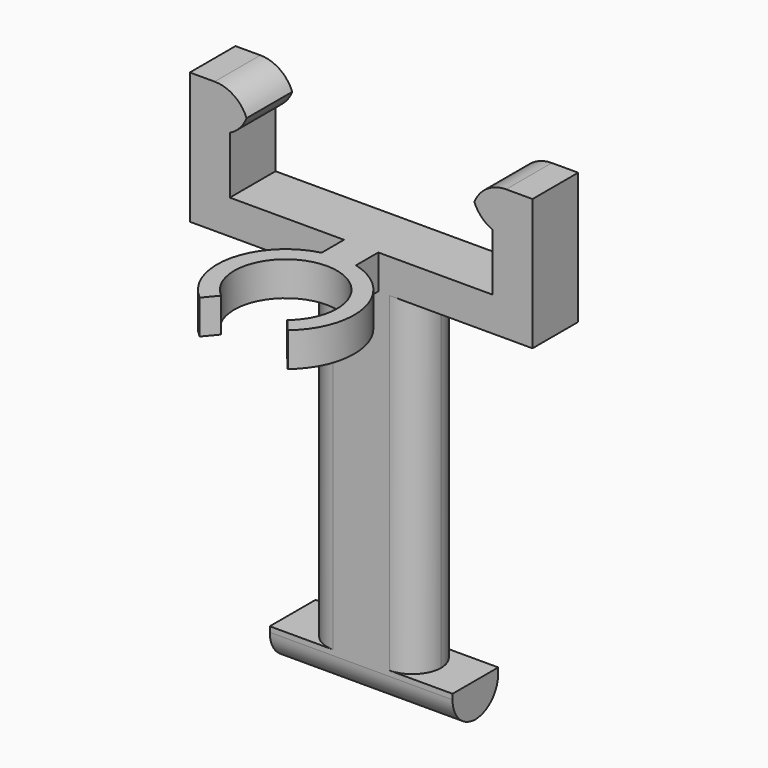
from build123d import *

# Parameters (mm, degrees)
F1_DEPTH    = 3
F3_DEPTH    = 5
F4_T1_DEPTH = 20
F4_T3_DEPTH = 18.7590602534
F4_T5_DEPTH = 18.4414894703
F5_T1_DEPTH = 28.8976125792
F5_T3_DEPTH = 28.7


# Not quite as in the source:
# - a fillet or chamfer that OpenCascade refuses, or shapes differently, is made with other operations: its cross-section is extruded or revolved along the edge and cut away or added


with BuildPart() as f1:
    # F0 (on Top) → F1 (new body)
    with BuildSketch(Plane.XY):
        with BuildLine():
            ThreePointArc((-2.8925442436, -3.447199994), (0, 4.5), (2.8925442436, -3.447199994))
            Line((2.8925442436, -3.447199994), (3.8567256581, -4.5962666587))
            ThreePointArc((3.8567256581, -4.5962666587), (5.9714768944, 0.5843489538), (2.8925442436, 5.2567278605))
            ThreePointArc((2.8925442436, 5.2567278605), (2.2135929139, 5.5767379723), (1.5, 5.8094750193))
            Line((1.5, 5.8094750193), (1.5, 8.2567278605))
            Line((1.5, 8.2567278605), (-1.5, 8.2567278605))
            Line((-1.5, 8.2567278605), (-1.5, 5.8094750193))
            ThreePointArc((-1.5, 5.8094750193), (-5.8517939481, 1.3253330104), (-3.8567256581, -4.5962666587))
            Line((-3.8567256581, -4.5962666587), (-2.8925442436, -3.447199994))
        make_face()
    extrude(amount=F1_DEPTH)

    # F2 (on face) → F3 (join)
    with BuildSketch(Plane(origin=(0, 8.2567278605, 0), x_dir=(-1, 0, 0), z_dir=(0, 1, 0))):
        Polygon((-15, 0), (-5, 0), (-5, -28.8976125792), (-8, -28.8976125792), (-8, -31.8976125792), (8, -31.8976125792), (8, -28.8976125792), (5, -28.8976125792), (5, 0), (15, 0), (15, 3), (15, 8), (15, 11.5052), (9.8263609009, 11.5052), (9.8263609009, 8), (11.4948, 8), (11.4948, 3), (0, 3), (-11.4948, 3), (-11.4948, 8), (-9.6895930523, 8), (-9.6895930523, 11.5052), (-13.1947930523, 11.5052), (-15, 11.5052), (-15, 8), (-15, 3), align=None)
    extrude(amount=F3_DEPTH)

    # F4: fillet of radius 3 on 4 edges, made by hand

    # F4_s2 → F4_t1 (cut)
    with BuildSketch(Plane.XZ.offset(-20.7567278605)):
        with BuildLine():
            ThreePointArc((12.6895930523, 11.5052), (10.5682727087, 10.6265203436), (9.6895930523, 8.5052))
            Line((9.6895930523, 8.5052), (9.6895930523, 11.5052))
            Line((9.6895930523, 11.5052), (12.6895930523, 11.5052))
        make_face()
        with BuildLine():
            ThreePointArc((-9.8263609009, 8.5052), (-10.7050405574, 10.6265203436), (-12.8263609009, 11.5052))
            Line((-12.8263609009, 11.5052), (-9.8263609009, 11.5052))
            Line((-9.8263609009, 11.5052), (-9.8263609009, 8.5052))
        make_face()
    extrude(amount=F4_T1_DEPTH, mode=Mode.SUBTRACT)

    # F4_s4 → F4_t3 (cut)
    with BuildSketch(Plane.XZ.offset(-20.1362579871)):
        with BuildLine():
            ThreePointArc((9.6895930523, 10.7518120507), (10.1811693284, 9.1062694588), (11.4948, 8))
            Line((11.4948, 8), (9.6895930523, 8))
            Line((9.6895930523, 8), (9.6895930523, 10.7518120507))
        make_face()
    extrude(amount=F4_T3_DEPTH, mode=Mode.SUBTRACT)

    # F4_s6 → F4_t5 (cut)
    with BuildSketch(Plane.XZ.offset(-19.9774725956)):
        with BuildLine():
            ThreePointArc((-11.4948, 8), (-10.2773726013, 9.1063185489), (-9.8263609009, 10.6882978941))
            Line((-9.8263609009, 10.6882978941), (-9.8263609009, 8))
            Line((-9.8263609009, 8), (-11.4948, 8))
        make_face()
    extrude(amount=F4_T5_DEPTH, mode=Mode.SUBTRACT)

    # F5: fillet of radius 2.54 on 6 edges, made by hand

    # F5_s2 → F5_t1 (cut)
    with BuildSketch(Plane.XY.offset(-28.8976125792)):
        with BuildLine():
            ThreePointArc((5, 10.7167278605), (4.2560512242, 12.5127790847), (2.46, 13.2567278605))
            Line((2.46, 13.2567278605), (5, 13.2567278605))
            Line((5, 13.2567278605), (5, 10.7167278605))
        make_face()
        with BuildLine():
            ThreePointArc((5, 10.7967278605), (4.2560512242, 9.0006766362), (2.46, 8.2567278605))
            Line((2.46, 8.2567278605), (5, 8.2567278605))
            Line((5, 8.2567278605), (5, 10.7967278605))
        make_face()
        with BuildLine():
            ThreePointArc((-2.46, 8.2567278605), (-4.2560512242, 9.0006766362), (-5, 10.7967278605))
            Line((-5, 10.7967278605), (-5, 8.2567278605))
            Line((-5, 8.2567278605), (-2.46, 8.2567278605))
        make_face()
        with BuildLine():
            ThreePointArc((-2.46, 13.2567278605), (-4.2560512242, 12.5127790847), (-5, 10.7167278605))
            Line((-5, 10.7167278605), (-5, 13.2567278605))
            Line((-5, 13.2567278605), (-2.46, 13.2567278605))
        make_face()
    extrude(amount=F5_T1_DEPTH, mode=Mode.SUBTRACT)

    # F5_s4 → F5_t3 (cut)
    with BuildSketch(Plane.YZ.offset(-14.35)):
        with BuildLine():
            ThreePointArc((8.2567278605, -29.3576125792), (9.0006766362, -31.1536638034), (10.7967278605, -31.8976125792))
            Line((10.7967278605, -31.8976125792), (8.2567278605, -31.8976125792))
            Line((8.2567278605, -31.8976125792), (8.2567278605, -29.3576125792))
        make_face()
        with BuildLine():
            ThreePointArc((13.2567278605, -29.3576125792), (12.5127790847, -31.1536638034), (10.7167278605, -31.8976125792))
            Line((10.7167278605, -31.8976125792), (13.2567278605, -31.8976125792))
            Line((13.2567278605, -31.8976125792), (13.2567278605, -29.3576125792))
        make_face()
    extrude(amount=F5_T3_DEPTH, mode=Mode.SUBTRACT)


solid = f1.part
